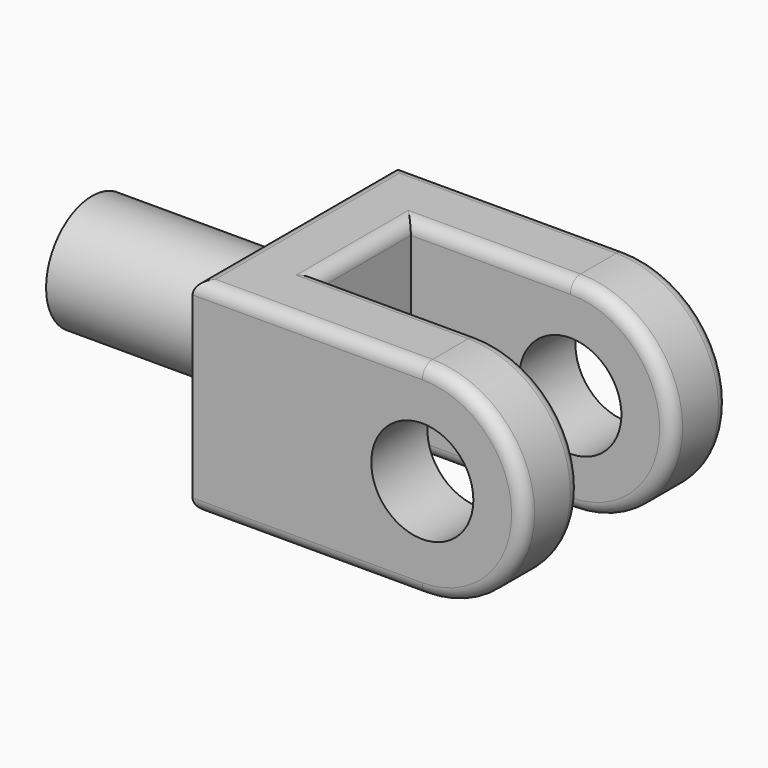
from build123d import *

# Parameters (mm, degrees)
F0_W      = 40
F0_H      = 32
F1_DEPTH  = 11
F3_DEPTH  = 11
F4_R      = 8
F5_DEPTH  = 76.2
F7_DEPTH  = 11
F8_R      = 8
F9_DEPTH  = 76.2
F10_R     = 2
F11_R     = 9
F12_DEPTH = 32
F13_R     = 8
F14_DEPTH = 36.068


with BuildPart() as f1:
    # F0 (on Right) → F1 (new body)
    with BuildSketch(Plane.YZ):
        with Locations((-0.2878075466, 20.7610073336)):
            Rectangle(F0_W, F0_H)
    extrude(amount=F1_DEPTH)

    # F2 (on face) → F3 (join)
    with BuildSketch(Plane.XZ.offset(20.2878075466)):
        with BuildLine():
            Line((11, 36.7610073336), (11, 4.7610073336))
            Line((11, 4.7610073336), (36, 4.7610073336))
            ThreePointArc((36, 4.7610073336), (52, 20.7610073336), (36, 36.7610073336))
            Line((36, 36.7610073336), (11, 36.7610073336))
        make_face()
    extrude(amount=-F3_DEPTH)

    # F4 (on face) → F5 (cut)
    with BuildSketch(Plane.XZ.offset(20.2878075466)):
        with Locations((36, 20.7610073336)):
            Circle(F4_R)
    extrude(amount=-F5_DEPTH, mode=Mode.SUBTRACT)

    # F6 (on face) → F7 (join)
    with BuildSketch(Plane(origin=(0, 19.7121924534, 0), x_dir=(-1, 0, 0), z_dir=(0, 1, 0))):
        with BuildLine():
            Line((-11, 4.7610073336), (-11, 36.7610073336))
            Line((-11, 36.7610073336), (-36, 36.7610073336))
            ThreePointArc((-36, 36.7610073336), (-52, 20.7610073336), (-36, 4.7610073336))
            Line((-36, 4.7610073336), (-11, 4.7610073336))
        make_face()
    extrude(amount=-F7_DEPTH)

    # F8 (on face) → F9 (cut)
    with BuildSketch(Plane(origin=(0, 19.7121924534, 0), x_dir=(-1, 0, 0), z_dir=(0, 1, 0))):
        with Locations((-36, 20.7610073336)):
            Circle(F8_R)
    extrude(amount=-F9_DEPTH, mode=Mode.SUBTRACT)

    # F10
    f10_edges = [f1.edges().sort_by_distance(p)[0] for p in [
        (36, 14.212192, 36.761007),
        (36, 14.212192, 4.761007),
        (52, 19.712192, 20.761007),
        (52, 8.712192, 20.761007),
        (36, -14.787808, 4.761007),
        (36, -14.787808, 36.761007),
        (52, -20.287808, 20.761007),
        (52, -9.287808, 20.761007),
        (18, 19.712192, 36.761007),
        (23.5, 8.712192, 36.761007),
        (11, -0.287808, 36.761007),
        (23.5, -9.287808, 36.761007),
        (18, -20.287808, 36.761007),
        (0, -0.287808, 36.761007),
        (18, -20.287808, 4.761007),
        (23.5, -9.287808, 4.761007),
        (11, -0.287808, 4.761007),
        (23.5, 8.712192, 4.761007),
        (18, 19.712192, 4.761007),
        (0, -0.287808, 4.761007),
    ]]
    fillet(f10_edges, radius=F10_R)

    # F11 (on face) → F12 (join)
    with BuildSketch(Plane(origin=(0, 0, 0), x_dir=(0, -1, 0), z_dir=(-1, 0, 0))):
        with Locations((0, 20.7610073336)):
            Circle(F11_R)
    extrude(amount=F12_DEPTH)

    # F13 (on face) → F14 (cut)
    with BuildSketch(Plane(origin=(0, 19.7121924534, 0), x_dir=(-1, 0, 0), z_dir=(0, 1, 0))):
        with Locations((-36, 20.7610073336)):
            Circle(F13_R)
    extrude(amount=-F14_DEPTH, mode=Mode.SUBTRACT)


solid = f1.part
